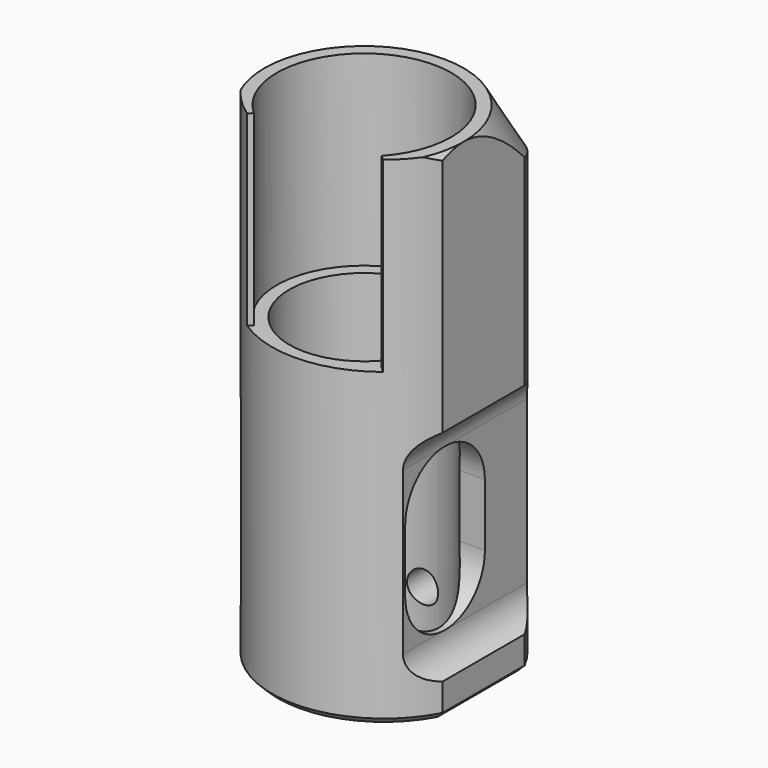
from build123d import *

# Parameters (mm, degrees)
F0_R      = 6
F1_DEPTH  = 40
F3_DEPTH  = 15
F6_SIZE   = 0.5
F8_DEPTH  = 16.0010001
F9_R      = 1.25
F10_DEPTH = 4.1326528028
F11_DEPTH = 15


# Not quite as in the source:
# - a feature names something its author has since deleted; it is built from what else it names


with BuildPart() as f1:
    # F0 (on Top) → F1 (new body)
    with BuildSketch(Plane.XY):
        with BuildLine():
            Line((-8, 6.1231056256), (-8, -2.1231056256))
            ThreePointArc((-8, -2.1231056256), (0, -7), (8, -2.1231056256))
            Line((8, -2.1231056256), (8, 6.1231056256))
            ThreePointArc((8, 6.1231056256), (6.1160859286, 8.6025368544), (3.5, 10.2915619759))
            Line((3.5, 10.2915619759), (3.5, 10))
            Line((3.5, 10), (-3.5, 10))
            Line((-3.5, 10), (-3.5, 10.2915619759))
            ThreePointArc((-3.5, 10.2915619759), (-6.1160859286, 8.6025368544), (-8, 6.1231056256))
        make_face()
        Circle(F0_R, mode=Mode.SUBTRACT)
    extrude(amount=F1_DEPTH)

    # F2 (on face) → F3 (cut)
    with BuildSketch(Plane.XY.offset(40)):
        with BuildLine():
            ThreePointArc((5.1812656518, -4.7068552395), (6.5295045586, -2.5230081686), (7, 0))
            ThreePointArc((7, 0), (-2.8330207662, 6.4010931362), (-4.7068552395, -5.1812656518))
            Line((-4.7068552395, -5.1812656518), (-4.0344473482, -4.4410848444))
            ThreePointArc((-4.0344473482, -4.4410848444), (-2.4283035139, 5.4866512596), (6, 0))
            ThreePointArc((6, 0), (5.5967181931, -2.1625784302), (4.4410848444, -4.0344473482))
            Line((4.4410848444, -4.0344473482), (5.1812656518, -4.7068552395))
        make_face()
        with BuildLine():
            Line((-4.0344473482, -4.4410848444), (-4.7068552395, -5.1812656518))
            ThreePointArc((-4.7068552395, -5.1812656518), (-2.523008134, -6.529504572), (7.42e-08, -7))
            ThreePointArc((7.42e-08, -7), (2.8330208001, -6.4010931212), (5.1812656518, -4.7068552395))
            Line((5.1812656518, -4.7068552395), (4.4410848444, -4.0344473482))
            ThreePointArc((4.4410848444, -4.0344473482), (0.2875361311, -5.9931062875), (-4.0344473482, -4.4410848444))
        make_face()
        with BuildLine():
            ThreePointArc((7.42e-08, -7), (-2.523008134, -6.529504572), (-4.7068552395, -5.1812656518))
            Line((-4.7068552395, -5.1812656518), (-4.9883233954, -5.4911033702))
            ThreePointArc((-4.9883233954, -5.4911033702), (-2.6057694927, -6.6145206106), (7.42e-08, -7))
        make_face()
        with BuildLine():
            Line((5.5754867215, -5.0649803835), (5.1812656518, -4.7068552395))
            ThreePointArc((5.1812656518, -4.7068552395), (2.8330208001, -6.4010931212), (7.42e-08, -7))
            ThreePointArc((7.42e-08, -7), (2.9508623284, -6.5024944292), (5.5754867215, -5.0649803835))
        make_face()
    extrude(amount=-F3_DEPTH, mode=Mode.SUBTRACT)

    # F4 (on Front) → F5 (revolve, cut)
    with BuildSketch(Plane.XZ):
        Polygon((0, 44.0566428006), (8, 40), (14.6664504582, 28.4533691002), (14.6664504582, 47.2484640777), (0, 47.2484640777), align=None)
    revolve(axis=Axis((0, 0, 27), (0, 0, 1)), mode=Mode.SUBTRACT)

    # F6
    f6_edges = [f1.edges().sort_by_distance(p)[0] for p in [
        (6.116086, 8.602537, 0),
        (-6.116086, 8.602537, 0),
        (-8, 2, 0),
        (0, -7, 0),
        (8, 2, 0),
    ]]
    chamfer(f6_edges, length=F6_SIZE)

    # F7 (on face) → F8 (cut, through all)
    with BuildSketch(Plane(origin=(-8, 0, 0), x_dir=(0, -1, 0), z_dir=(-1, 0, 0))):
        with BuildLine():
            ThreePointArc((2.1231056256, 5.6099524336), (3.4994587083, 7.0625303231), (4, 9))
            ThreePointArc((4, 9), (3.7742546282, 10.3247648854), (3.1224989992, 11.5))
            ThreePointArc((3.1224989992, 11.5), (2.6602891079, 11.0128840226), (2.1231056256, 10.6099524336))
            Line((2.1231056256, 10.6099524336), (2.1231056256, 5.6099524336))
        make_face()
        with BuildLine():
            ThreePointArc((3.1224989992, 11.5), (3.7742546282, 10.3247648854), (4, 9))
            Line((4, 9), (4, 14))
            ThreePointArc((4, 14), (3.7742546282, 12.6752351146), (3.1224989992, 11.5))
        make_face()
        with BuildLine():
            ThreePointArc((2.1231056256, 10.6099524336), (2.6602891079, 11.0128840226), (3.1224989992, 11.5))
            ThreePointArc((3.1224989992, 11.5), (2.6602891079, 11.9871159774), (2.1231056256, 12.3900475664))
            Line((2.1231056256, 12.3900475664), (2.1231056256, 10.6099524336))
        make_face()
        with BuildLine():
            ThreePointArc((2.1231056256, 12.3900475664), (2.6602891079, 11.9871159774), (3.1224989992, 11.5))
            ThreePointArc((3.1224989992, 11.5), (3.7742546282, 12.6752351146), (4, 14))
            ThreePointArc((4, 14), (3.4994587083, 15.9374696769), (2.1231056256, 17.3900475664))
            Line((2.1231056256, 17.3900475664), (2.1231056256, 12.3900475664))
        make_face()
        with BuildLine():
            ThreePointArc((-4, 9), (-1.9374696769, 5.5005412917), (2.1231056256, 5.6099524336))
            Line((2.1231056256, 5.6099524336), (2.1231056256, 10.6099524336))
            ThreePointArc((2.1231056256, 10.6099524336), (-0.66913597, 10.0563649949), (-3.1224989992, 11.5))
            ThreePointArc((-3.1224989992, 11.5), (-3.7742546282, 10.3247648854), (-4, 9))
        make_face()
        with BuildLine():
            Line((2.1231056256, 10.6099524336), (2.1231056256, 12.3900475664))
            ThreePointArc((2.1231056256, 12.3900475664), (-0.66913597, 12.9436350051), (-3.1224989992, 11.5))
            ThreePointArc((-3.1224989992, 11.5), (-0.66913597, 10.0563649949), (2.1231056256, 10.6099524336))
        make_face()
        with BuildLine():
            ThreePointArc((-3.1224989992, 11.5), (-0.66913597, 12.9436350051), (2.1231056256, 12.3900475664))
            Line((2.1231056256, 12.3900475664), (2.1231056256, 17.3900475664))
            ThreePointArc((2.1231056256, 17.3900475664), (-1.9374696769, 17.4994587083), (-4, 14))
            ThreePointArc((-4, 14), (-3.7742546282, 12.6752351146), (-3.1224989992, 11.5))
        make_face()
        with BuildLine():
            Line((-4, 14), (-4, 9))
            ThreePointArc((-4, 9), (-3.7742546282, 10.3247648854), (-3.1224989992, 11.5))
            ThreePointArc((-3.1224989992, 11.5), (-3.7742546282, 12.6752351146), (-4, 14))
        make_face()
    extrude(amount=-F8_DEPTH, mode=Mode.SUBTRACT)

    # F9 (on face) → F10 (cut, through all)
    with BuildSketch(Plane(origin=(0, 10, 0), x_dir=(-1, 0, 0), z_dir=(0, 1, 0))):
        with Locations((0, 3.5)):
            Circle(F9_R)
        with Locations((0, 22)):
            Circle(F9_R)
        with Locations((0, 27)):
            Circle(F9_R)
        with Locations((0, 32)):
            Circle(F9_R)
    extrude(amount=-F10_DEPTH, mode=Mode.SUBTRACT)

    # F9 (on face) → F11 (cut)
    with BuildSketch(Plane(origin=(0, 10, 0), x_dir=(-1, 0, 0), z_dir=(0, 1, 0))):
        with BuildLine():
            ThreePointArc((-6.5, 18), (-7.232233047, 19.767766953), (-9, 20.5))
            Line((-9, 20.5), (-9.5, 20.5))
            Line((-9.5, 20.5), (-9.5, 2.5))
            Line((-9.5, 2.5), (-9, 2.5))
            ThreePointArc((-9, 2.5), (-7.232233047, 3.232233047), (-6.5, 5))
            Line((-6.5, 5), (-6.5, 18))
        make_face()
        with BuildLine():
            Line((10.5, 20.5), (9, 20.5))
            ThreePointArc((9, 20.5), (7.232233047, 19.767766953), (6.5, 18))
            Line((6.5, 18), (6.5, 5))
            ThreePointArc((6.5, 5), (7.232233047, 3.232233047), (9, 2.5))
            Line((9, 2.5), (10.5, 2.5))
            Line((10.5, 2.5), (10.5, 20.5))
        make_face()
    extrude(amount=-F11_DEPTH, mode=Mode.SUBTRACT)


solid = f1.part
